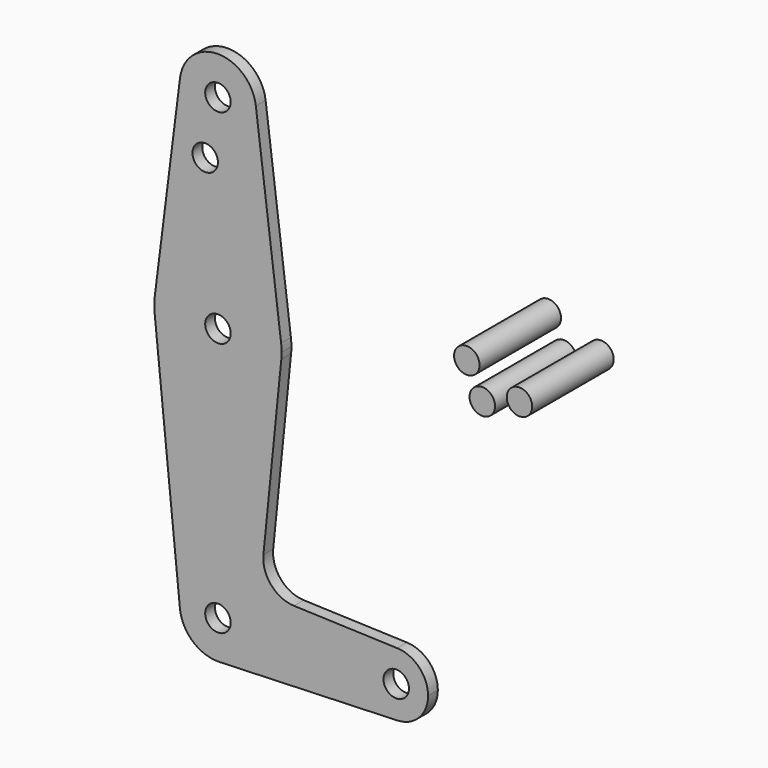
from build123d import *

# Parameters (mm, degrees)
F0_R     = 3.175
F1_DEPTH = 3.048
F2_R     = 3.175
F3_DEPTH = 12.7
F5_R     = 3.175
F6_DEPTH = 12.7
F4_R     = 3.175
F7_DEPTH = 12.7


# Not quite as in the source:
# - ends of sketch curves that miss each other by under 0.0002 mm in the source are joined


with BuildPart() as f1:
    # F0 (on Front) → F1 (new body)
    with BuildSketch(Plane.XZ):
        with BuildLine():
            ThreePointArc((-60.2516630306, 53.6090369056), (-51.3927330128, 42.919997736), (-41.2753472159, 52.4265588422))
            ThreePointArc((-41.2753472159, 52.4265588422), (-41.2940423216, 53.0230420842), (-41.3500542517, 53.6171838422))
            ThreePointArc((-41.3500542517, 53.6171838422), (-50.8044526635, 61.9515579575), (-60.2516630306, 53.6090369056))
        make_face()
        with Locations((-50.8003472159, 52.4265588422)):
            Circle(F0_R, mode=Mode.SUBTRACT)
        with BuildLine():
            ThreePointArc((-41.3500542517, 53.6171838422), (-41.2940423216, 53.0230420842), (-41.2753472159, 52.4265588422))
            ThreePointArc((-41.2753472159, 52.4265588422), (-51.3927330128, 42.919997736), (-60.2516630306, 53.6090369056))
            Line((-60.2516630306, 53.6090369056), (-66.5508354393, 3.6109342409))
            ThreePointArc((-66.5508354393, 3.6109342409), (-50.800347015, 17.5015588422), (-35.0498589422, 3.6109338422))
            Line((-35.0498589422, 3.6109338422), (-41.3500542517, 53.6171838422))
        make_face()
        with Locations((-53.9753472159, 38.1517588422)):
            Circle(F0_R, mode=Mode.SUBTRACT)
        with BuildLine():
            ThreePointArc((-34.9253472159, 1.6265588422), (-34.9565057255, 2.6206975789), (-35.0498589422, 3.6109338422))
            ThreePointArc((-35.0498589422, 3.6109338422), (-50.800347015, 17.5015588422), (-66.5508354393, 3.6109342409))
            ThreePointArc((-66.5508354393, 3.6109342409), (-66.6740910318, 1.8262642914), (-66.5957727323, 0.0390583677))
            ThreePointArc((-66.5957727323, 0.0390583677), (-50.8003466117, -14.2484411578), (-35.0049215787, 0.03905957))
            ThreePointArc((-35.0049215787, 0.03905957), (-34.9452532869, 0.8318126534), (-34.9253472159, 1.6265588422))
        make_face()
        with Locations((-50.8003472159, 1.6265588422)):
            Circle(F0_R, mode=Mode.SUBTRACT)
        with BuildLine():
            ThreePointArc((-35.0049215787, 0.03905957), (-50.8003466117, -14.2484411578), (-66.5957727323, 0.0390583677))
            Line((-66.5957727323, 0.0390583677), (-60.2776025543, -62.8259411578))
            ThreePointArc((-60.2776025543, -62.8259411578), (-51.2771951483, -52.3603848114), (-41.2753472159, -61.8734411578))
            ThreePointArc((-41.2753472159, -61.8734411578), (-43.9459387338, -68.4872682919), (-50.460168079, -71.3923645819))
            Line((-50.460168079, -71.3923645819), (-6.066865073, -69.8058773614))
            ThreePointArc((-6.066865073, -69.8058773614), (-14.2878472159, -61.8734411578), (-6.066865073, -53.9410049541))
            Line((-6.066865073, -53.9410049541), (-31.8327472154, -53.0202074469))
            ThreePointArc((-31.8327472154, -53.0202074469), (-37.5391473185, -50.3020820079), (-39.4591606236, -44.2800593454))
            Line((-39.4591606236, -44.2800593454), (-35.0049215787, 0.03905957))
        make_face()
        with BuildLine():
            ThreePointArc((-41.2753472159, -61.8734411578), (-51.2771951483, -52.3603848114), (-60.2776025543, -62.8259411578))
            ThreePointArc((-60.2776025543, -62.8259411578), (-57.0627303844, -69.0503612528), (-50.460168079, -71.3923645819))
            ThreePointArc((-50.460168079, -71.3923645819), (-43.9459387338, -68.4872682919), (-41.2753472159, -61.8734411578))
        make_face()
        with Locations((-50.8003472159, -61.8734411578)):
            Circle(F0_R, mode=Mode.SUBTRACT)
        with BuildLine():
            ThreePointArc((-6.066865073, -53.9410049541), (-14.2878472159, -61.8734411578), (-6.066865073, -69.8058773614))
            ThreePointArc((-6.066865073, -69.8058773614), (-0.6383403112, -67.3849639392), (1.5871527841, -61.8734411578))
            ThreePointArc((1.5871527841, -61.8734411578), (-0.6383403112, -56.3619183763), (-6.066865073, -53.9410049541))
        make_face()
        with Locations((-6.3503472159, -61.8734411578)):
            Circle(F0_R, mode=Mode.SUBTRACT)
    extrude(amount=F1_DEPTH)


with BuildPart() as f3:
    # F2 (on Front) → F3 (new body, symmetric)
    with BuildSketch(Plane.XZ):
        with Locations((18.9683057667, 21.2909408399)):
            Circle(F2_R)
    extrude(amount=F3_DEPTH, both=True)


with BuildPart() as f6:
    # F5 (on Front) → F6 (new body, symmetric)
    with BuildSketch(Plane.XZ):
        with Locations((32.1025885642, 16.4576992393)):
            Circle(F5_R)
    extrude(amount=F6_DEPTH, both=True)


with BuildPart() as f7:
    # F4 (on Front) → F7 (new body, symmetric)
    with BuildSketch(Plane.XZ):
        with Locations((22.8300068826, 13.5314479956)):
            Circle(F4_R)
    extrude(amount=F7_DEPTH, both=True)


solid = Compound([f1.part, f3.part, f6.part, f7.part])
